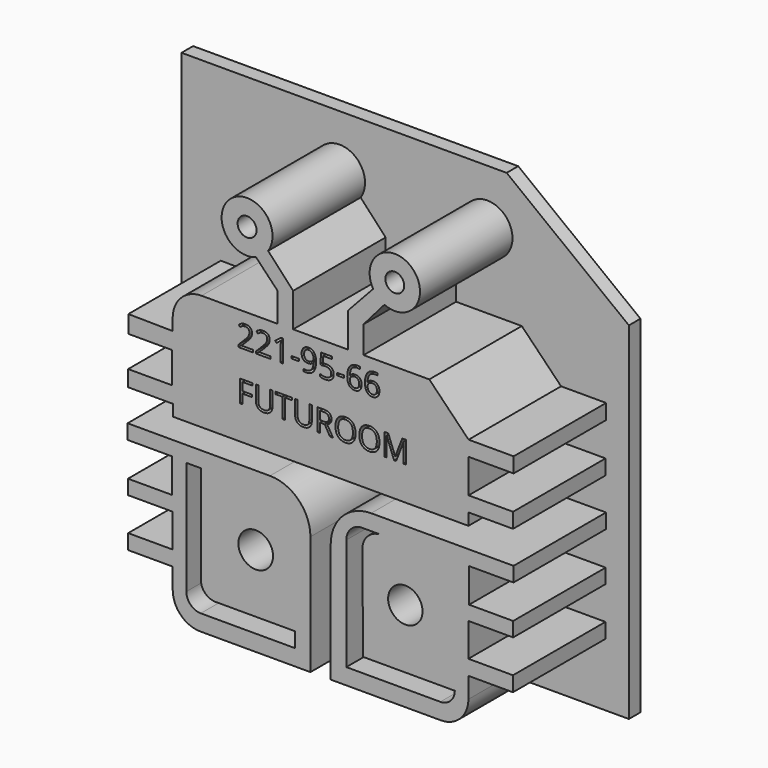
from build123d import *

# Parameters (mm, degrees)
F0_R           = 1.1991628377
F1_DEPTH       = 8
F0_R_2         = 0.6541163762
F0_R_3         = 0.651723112
F0_R_4         = 1.1913062279
F2_DEPTH       = 8
F4_DEPTH       = 1
F5_TEXT_SIZE   = 2.1452034591
F5_TEXT_SIZE_2 = 2.1230966215
F6_DEPTH       = 3


# Not quite as in the source:
# - Text() gives the source's letters only with a copy of the font that has no kerning and outlines rounded to 1/6400 em; it was checked with that copy


with BuildPart() as f1:
    # F0 (on Front) → F1 (new body)
    with BuildSketch(Plane.XZ):
        with BuildLine():
            Line((-5.0600913255, -10.4540819302), (-14.9129647762, -10.4540819302))
            Line((-14.9129647762, -10.4540819302), (-14.9129647762, -11.4703048021))
            Line((-14.9129647762, -11.4703048021), (-11.8368314579, -11.4703048021))
            Line((-11.8368314579, -11.4703048021), (-11.8368314579, -13.8218998909))
            Line((-11.8368314579, -13.8218998909), (-14.8851303384, -13.8218998909))
            Line((-14.8851303384, -13.8218998909), (-14.8851303384, -14.825752005))
            Line((-14.8851303384, -14.825752005), (-11.7872171104, -14.825752005))
            Line((-11.7872171104, -14.825752005), (-11.7872171104, -17.1329826117))
            Line((-11.7872171104, -17.1329826117), (-14.8721681908, -17.1329826117))
            Line((-14.8721681908, -17.1329826117), (-14.8721681908, -18.1699413806))
            Line((-14.8721681908, -18.1699413806), (-11.7872171104, -18.1699413806))
            Line((-11.7872171104, -18.1699413806), (-11.7872171104, -19.601172334))
            ThreePointArc((-11.7872171104, -19.601172334), (-11.2307199946, -20.9446752182), (-9.8872171104, -21.501172334))
            Line((-9.8872171104, -21.501172334), (-2.2600913255, -21.501172334))
            Line((-2.2600913255, -21.501172334), (-2.2600913255, -13.2540819302))
            ThreePointArc((-2.2600913255, -13.2540819302), (-3.0801923381, -11.2741829429), (-5.0600913255, -10.4540819302))
        make_face()
        with BuildLine():
            Line((-10.8474520966, -19.3861606861), (-10.8474520966, -11.5441279486))
            Line((-10.8474520966, -11.5441279486), (-9.8374737427, -11.5441279486))
            Line((-9.8374737427, -11.5441279486), (-4.4398872652, -11.5441279486))
            ThreePointArc((-4.4398872652, -11.5441279486), (-3.6620698059, -11.8663104893), (-3.3398872652, -12.6441279486))
            Line((-3.3398872652, -12.6441279486), (-3.3398872652, -19.3554535508))
            Line((-3.3398872652, -19.3554535508), (-3.3398872652, -20.3861606861))
            Line((-3.3398872652, -20.3861606861), (-9.8474520966, -20.3861606861))
            ThreePointArc((-9.8474520966, -20.3861606861), (-10.5545588778, -20.0932674673), (-10.8474520966, -19.3861606861))
        make_face(mode=Mode.SUBTRACT)
        with BuildLine():
            Line((-4.4398872652, -11.5441279486), (-9.8374737427, -11.5441279486))
            Line((-9.8374737427, -11.5441279486), (-9.8374737427, -18.3554535508))
            ThreePointArc((-9.8374737427, -18.3554535508), (-9.5445805239, -19.062560332), (-8.8374737427, -19.3554535508))
            Line((-8.8374737427, -19.3554535508), (-3.3398872652, -19.3554535508))
            Line((-3.3398872652, -19.3554535508), (-3.3398872652, -12.6441279486))
            ThreePointArc((-3.3398872652, -12.6441279486), (-3.6620698059, -11.8663104893), (-4.4398872652, -11.5441279486))
        make_face()
        with Locations((-6.0443845578, -15.2789726853)):
            Circle(F0_R, mode=Mode.SUBTRACT)
    extrude(amount=F1_DEPTH)

    # F0 (on Front) → F2, piece 2 (join)
    with BuildSketch(Plane.XZ):
        with BuildLine():
            Line((-5.0600913255, -10.4540819302), (-14.9129647762, -10.4540819302))
            Line((-14.9129647762, -10.4540819302), (-14.9129647762, -11.4703048021))
            Line((-14.9129647762, -11.4703048021), (-11.8368314579, -11.4703048021))
            Line((-11.8368314579, -11.4703048021), (-11.8368314579, -13.8218998909))
            Line((-11.8368314579, -13.8218998909), (-14.8851303384, -13.8218998909))
            Line((-14.8851303384, -13.8218998909), (-14.8851303384, -14.825752005))
            Line((-14.8851303384, -14.825752005), (-11.7872171104, -14.825752005))
            Line((-11.7872171104, -14.825752005), (-11.7872171104, -17.1329826117))
            Line((-11.7872171104, -17.1329826117), (-14.8721681908, -17.1329826117))
            Line((-14.8721681908, -17.1329826117), (-14.8721681908, -18.1699413806))
            Line((-14.8721681908, -18.1699413806), (-11.7872171104, -18.1699413806))
            Line((-11.7872171104, -18.1699413806), (-11.7872171104, -19.601172334))
            ThreePointArc((-11.7872171104, -19.601172334), (-11.2307199946, -20.9446752182), (-9.8872171104, -21.501172334))
            Line((-9.8872171104, -21.501172334), (-2.2600913255, -21.501172334))
            Line((-2.2600913255, -21.501172334), (-2.2600913255, -13.2540819302))
            ThreePointArc((-2.2600913255, -13.2540819302), (-3.0801923381, -11.2741829429), (-5.0600913255, -10.4540819302))
        make_face()
        with BuildLine():
            Line((-10.8474520966, -19.3861606861), (-10.8474520966, -11.5441279486))
            Line((-10.8474520966, -11.5441279486), (-9.8374737427, -11.5441279486))
            Line((-9.8374737427, -11.5441279486), (-4.4398872652, -11.5441279486))
            ThreePointArc((-4.4398872652, -11.5441279486), (-3.6620698059, -11.8663104893), (-3.3398872652, -12.6441279486))
            Line((-3.3398872652, -12.6441279486), (-3.3398872652, -19.3554535508))
            Line((-3.3398872652, -19.3554535508), (-3.3398872652, -20.3861606861))
            Line((-3.3398872652, -20.3861606861), (-9.8474520966, -20.3861606861))
            ThreePointArc((-9.8474520966, -20.3861606861), (-10.5545588778, -20.0932674673), (-10.8474520966, -19.3861606861))
        make_face(mode=Mode.SUBTRACT)
    extrude(amount=F2_DEPTH)



with BuildPart() as f1b:
    # F0 (on Front) → F1, piece 2 (new body)
    with BuildSketch(Plane.XZ):
        with BuildLine():
            Line((-11.7916371673, -3.8222426083), (-14.8589555174, -3.7834849209))
            Line((-14.8589555174, -3.7834849209), (-14.8589555174, -4.9919658341))
            Line((-14.8589555174, -4.9919658341), (-11.8359290063, -4.9919658341))
            Line((-11.8359290063, -4.9919658341), (-11.8359290063, -7.1406057104))
            Line((-11.8359290063, -7.1406057104), (-14.8734524846, -7.1406057104))
            Line((-14.8734524846, -7.1406057104), (-14.8734524846, -8.2491952926))
            Line((-14.8734524846, -8.2491952926), (-11.755543761, -8.2491952926))
            Line((-11.755543761, -8.2491952926), (-11.755543761, -9.0344464406))
            Line((-11.755543761, -9.0344464406), (8.6731323972, -9.0344464406))
            Line((8.6731323972, -9.0344464406), (8.6731323972, -8.2123074681))
            Line((8.6731323972, -8.2123074681), (11.760010384, -8.2123074681))
            Line((11.760010384, -8.2123074681), (11.760010384, -7.1730306372))
            Line((11.760010384, -7.1730306372), (8.6838770658, -7.1730306372))
            Line((8.6838770658, -7.1730306372), (8.6838770658, -4.8247333616))
            Line((8.6838770658, -4.8247333616), (11.8012083694, -4.8247333616))
            Line((11.8012083694, -4.8247333616), (11.8012083694, -3.7810450885))
            Line((11.8012083694, -3.7810450885), (8.6838770658, -3.7810450885))
            Line((8.6838770658, -3.7810450885), (5.9647937305, -0.9932990652))
            Line((5.9647937305, -0.9932990652), (1.4192573726, -0.9932990652))
            Line((1.4192573726, -0.9932990652), (1.4192573726, 0.8880862151))
            Line((1.4192573726, 0.8880862151), (2.8611947782, 2.5497477036))
            ThreePointArc((2.8611947782, 2.5497477036), (4.7409001729, 5.4382086326), (2.0784286316, 3.2501171809))
            Line((2.0784286316, 3.2501171809), (0.3343709395, 1.3687321916))
            Line((0.3343709395, 1.3687321916), (0.3343709395, -1.0070313001))
            Line((0.3343709395, -1.0070313001), (-3.4558647312, -1.0070313001))
            Line((-3.4558647312, -1.0070313001), (-3.4558647312, 1.3412669068))
            Line((-3.4558647312, 1.3412669068), (-5.1861898974, 3.2089194283))
            ThreePointArc((-5.1861898974, 3.2089194283), (-7.7332725937, 5.5839635677), (-6.0238866135, 2.5497479364))
            Line((-6.0238866135, 2.5497479364), (-4.5407512225, 0.9979485767))
            Line((-4.5407512225, 0.9979485767), (-4.5407512225, -1.0207640007))
            Line((-4.5407512225, -1.0207640007), (-9.7916371673, -1.0207640007))
            ThreePointArc((-9.7916371673, -1.0207640007), (-11.2058507297, -1.6065504383), (-11.7916371673, -3.0207640007))
            Line((-11.7916371673, -3.0207640007), (-11.7916371673, -3.8222426083))
        make_face()
        with Locations((-6.6436350291, 4.1992164708)):
            Circle(F0_R_2, mode=Mode.SUBTRACT)
        with Locations((3.5783580142, 4.1388963762)):
            Circle(F0_R_3, mode=Mode.SUBTRACT)
    extrude(amount=F1_DEPTH)

    # F0 (on Front) → F2 (join)
    with BuildSketch(Plane.XZ):
        with BuildLine():
            Line((-11.7916371673, -3.8222426083), (-14.8589555174, -3.7834849209))
            Line((-14.8589555174, -3.7834849209), (-14.8589555174, -4.9919658341))
            Line((-14.8589555174, -4.9919658341), (-11.8359290063, -4.9919658341))
            Line((-11.8359290063, -4.9919658341), (-11.8359290063, -7.1406057104))
            Line((-11.8359290063, -7.1406057104), (-14.8734524846, -7.1406057104))
            Line((-14.8734524846, -7.1406057104), (-14.8734524846, -8.2491952926))
            Line((-14.8734524846, -8.2491952926), (-11.755543761, -8.2491952926))
            Line((-11.755543761, -8.2491952926), (-11.755543761, -9.0344464406))
            Line((-11.755543761, -9.0344464406), (8.6731323972, -9.0344464406))
            Line((8.6731323972, -9.0344464406), (8.6731323972, -8.2123074681))
            Line((8.6731323972, -8.2123074681), (11.760010384, -8.2123074681))
            Line((11.760010384, -8.2123074681), (11.760010384, -7.1730306372))
            Line((11.760010384, -7.1730306372), (8.6838770658, -7.1730306372))
            Line((8.6838770658, -7.1730306372), (8.6838770658, -4.8247333616))
            Line((8.6838770658, -4.8247333616), (11.8012083694, -4.8247333616))
            Line((11.8012083694, -4.8247333616), (11.8012083694, -3.7810450885))
            Line((11.8012083694, -3.7810450885), (8.6838770658, -3.7810450885))
            Line((8.6838770658, -3.7810450885), (5.9647937305, -0.9932990652))
            Line((5.9647937305, -0.9932990652), (1.4192573726, -0.9932990652))
            Line((1.4192573726, -0.9932990652), (1.4192573726, 0.8880862151))
            Line((1.4192573726, 0.8880862151), (2.8611947782, 2.5497477036))
            ThreePointArc((2.8611947782, 2.5497477036), (4.7409001729, 5.4382086326), (2.0784286316, 3.2501171809))
            Line((2.0784286316, 3.2501171809), (0.3343709395, 1.3687321916))
            Line((0.3343709395, 1.3687321916), (0.3343709395, -1.0070313001))
            Line((0.3343709395, -1.0070313001), (-3.4558647312, -1.0070313001))
            Line((-3.4558647312, -1.0070313001), (-3.4558647312, 1.3412669068))
            Line((-3.4558647312, 1.3412669068), (-5.1861898974, 3.2089194283))
            ThreePointArc((-5.1861898974, 3.2089194283), (-7.7332725937, 5.5839635677), (-6.0238866135, 2.5497479364))
            Line((-6.0238866135, 2.5497479364), (-4.5407512225, 0.9979485767))
            Line((-4.5407512225, 0.9979485767), (-4.5407512225, -1.0207640007))
            Line((-4.5407512225, -1.0207640007), (-9.7916371673, -1.0207640007))
            ThreePointArc((-9.7916371673, -1.0207640007), (-11.2058507297, -1.6065504383), (-11.7916371673, -3.0207640007))
            Line((-11.7916371673, -3.0207640007), (-11.7916371673, -3.8222426083))
        make_face()
        with Locations((-6.6436350291, 4.1992164708)):
            Circle(F0_R_2, mode=Mode.SUBTRACT)
        with Locations((3.5783580142, 4.1388963762)):
            Circle(F0_R_3, mode=Mode.SUBTRACT)
    extrude(amount=F2_DEPTH)


with BuildPart() as f1c:
    # F0 (on Front) → F1, piece 3 (new body)
    with BuildSketch(Plane.XZ):
        with BuildLine():
            Line((1.3332831969, -12.8544036871), (1.3846717935, -19.3554535508))
            Line((1.3846717935, -19.3554535508), (1.384914523, -19.3861606861))
            Line((1.384914523, -19.3861606861), (7.7304907425, -19.3861606861))
            Line((7.7304907425, -19.3861606861), (7.7304907425, -11.5441279486))
            Line((7.7304907425, -11.5441279486), (2.949451562, -11.5441279486))
            Line((2.949451562, -11.5441279486), (2.6332425844, -11.5441279486))
            ThreePointArc((2.6332425844, -11.5441279486), (1.7103778976, -11.928529363), (1.3332831969, -12.8544036871))
        make_face()
        with Locations((4.306727089, -15.2789726853)):
            Circle(F0_R_4, mode=Mode.SUBTRACT)
    extrude(amount=F1_DEPTH)

    # F0 (on Front) → F2, piece 3 (join)
    with BuildSketch(Plane.XZ):
        with BuildLine():
            Line((-0.8568700287, -13.2540819302), (-0.8568700287, -21.501172334))
            Line((-0.8568700287, -21.501172334), (6.7702557563, -21.501172334))
            ThreePointArc((6.7702557563, -21.501172334), (8.1137586405, -20.9446752182), (8.6702557563, -19.601172334))
            Line((8.6702557563, -19.601172334), (8.6702557563, -18.1699413806))
            Line((8.6702557563, -18.1699413806), (11.7552068367, -18.1699413806))
            Line((11.7552068367, -18.1699413806), (11.7552068367, -17.1329826117))
            Line((11.7552068367, -17.1329826117), (8.6702557563, -17.1329826117))
            Line((8.6702557563, -17.1329826117), (8.6702557563, -14.825752005))
            Line((8.6702557563, -14.825752005), (11.7681689842, -14.825752005))
            Line((11.7681689842, -14.825752005), (11.7681689842, -13.8218998909))
            Line((11.7681689842, -13.8218998909), (8.7198701038, -13.8218998909))
            Line((8.7198701038, -13.8218998909), (8.7198701038, -11.4703048021))
            Line((8.7198701038, -11.4703048021), (11.796003422, -11.4703048021))
            Line((11.796003422, -11.4703048021), (11.796003422, -10.4540819302))
            Line((11.796003422, -10.4540819302), (1.9431299713, -10.4540819302))
            ThreePointArc((1.9431299713, -10.4540819302), (-0.036769016, -11.2741829429), (-0.8568700287, -13.2540819302))
        make_face()
        with BuildLine():
            Line((0.2229259111, -20.3861606861), (0.2229259111, -19.3554535508))
            Line((0.2229259111, -19.3554535508), (0.2229259111, -12.6441279486))
            ThreePointArc((0.2229259111, -12.6441279486), (0.5451084518, -11.8663104893), (1.3229259111, -11.5441279486))
            Line((1.3229259111, -11.5441279486), (2.6332425844, -11.5441279486))
            Line((2.6332425844, -11.5441279486), (2.949451562, -11.5441279486))
            Line((2.949451562, -11.5441279486), (7.7304907425, -11.5441279486))
            Line((7.7304907425, -11.5441279486), (7.7304907425, -19.3861606861))
            ThreePointArc((7.7304907425, -19.3861606861), (7.4375975237, -20.0932674673), (6.7304907425, -20.3861606861))
            Line((6.7304907425, -20.3861606861), (0.2229259111, -20.3861606861))
        make_face(mode=Mode.SUBTRACT)
    extrude(amount=F2_DEPTH)


with BuildPart() as f1_1:
    add(f1.part)

    add(f1b.part)  # F4 merges F1b

    add(f1c.part)  # F4 merges F1c
    # F3 (on Front) → F4 (join)
    with BuildSketch(Plane.XZ):
        Polygon((-17.5797268748, 7.9955961555), (-17.5797268748, 7.2980159894), (-17.5797268748, -22.5235130638), (13.3753689006, -22.5235130638), (13.3753689006, 1.4557873365), (4.9172155559, 7.9955961555), align=None)
    extrude(amount=-F4_DEPTH)

    # F5 (on face) → F6 (cut)
    with BuildSketch(Plane.XZ.offset(8)):
        with Locations((-7.3484274574, -3.3201740523)):
            Text('221-95-66', F5_TEXT_SIZE, font='Open Sans', text_align=(TextAlign.LEFT, TextAlign.BOTTOM))
        with Locations((-7.3308889987, -6.7125959322)):
            Text('FUTUROOM', F5_TEXT_SIZE_2, font='Open Sans', text_align=(TextAlign.LEFT, TextAlign.BOTTOM))
    extrude(amount=-F6_DEPTH, mode=Mode.SUBTRACT)


with BuildPart() as f7_1:
    # F7: copy of F1
    add(f1_1.part)


solid = Compound([f1_1.part, f7_1.part])
